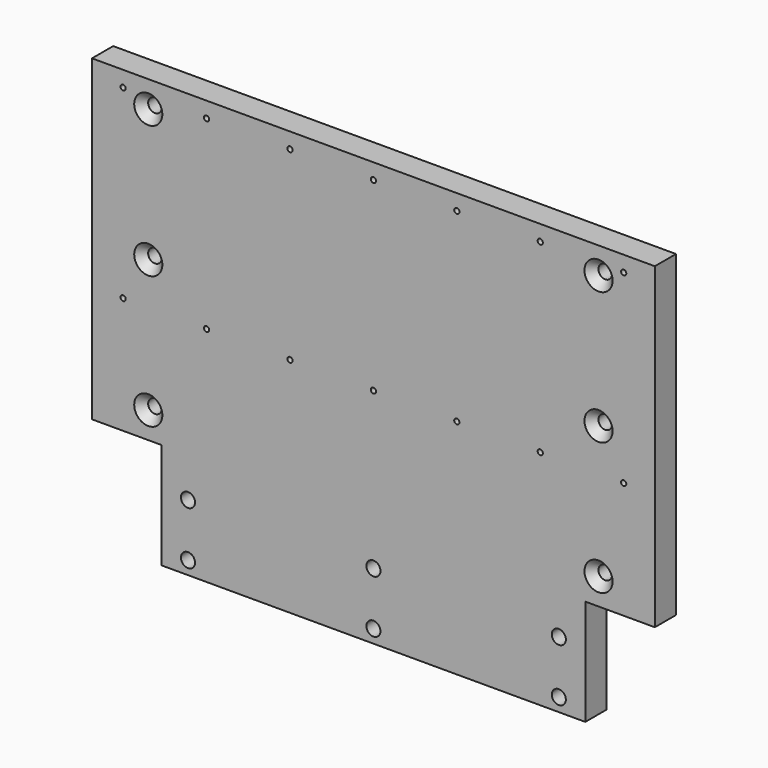
from build123d import *

# Parameters (mm, degrees)
F0_W           = 269.875
F0_H           = 203.2
F1_DEPTH       = 12.7
F2_W           = 33.3375
F2_H           = 50.8
F3_DEPTH       = 12.7
F5_D           = 6.7564
F7_D           = 2.5
F7_DEPTH       = 20.55
F7_TIP         = 0.7510757738
F9_D           = 6.5278
F9_CSINK_D     = 13.4874
F9_CSINK_ANGLE = 82


# Not quite as in the source:
# - a feature names something its author has since deleted; it is built from what else it names


with BuildPart() as f1:
    # F0 (on Front) → F1 (new body)
    with BuildSketch(Plane.XZ):
        with Locations((134.9375, 101.6)):
            Rectangle(F0_W, F0_H)
    extrude(amount=F1_DEPTH)

    # F2 (on face) → F3 (cut, through all)
    with BuildSketch(Plane.XZ.offset(12.7)):
        with Locations((16.66875, 25.4)):
            Rectangle(F2_W, F2_H)
        with Locations((253.20625, 25.4)):
            Rectangle(F2_W, F2_H)
    extrude(amount=-F3_DEPTH, mode=Mode.SUBTRACT)

    # F5 (through all)
    with Locations(Plane.XZ.offset(12.7)):
        with Locations((223.8375, 31.75), (223.8375, 6.35), (134.9375, 6.35), (134.9375, 31.75), (46.0375, 31.75), (46.0375, 6.35)):
            Hole(F5_D / 2)

    # F7
    with Locations(Plane.XZ.offset(12.7)):
        with Locations((54.9375, 195.7), (94.9375, 195.7), (134.9375, 195.7), (174.9375, 195.7), (214.9375, 195.7), (214.9375, 106.8), (174.9375, 106.8), (134.9375, 106.8), (94.9375, 106.8), (54.9375, 106.8), (14.9375, 195.7), (14.9375, 106.8), (254.9375, 195.7), (254.9375, 106.8)):
            Hole(F7_D / 2, depth=F7_DEPTH)
            with Locations((0, 0, -(F7_DEPTH + F7_TIP / 2))):  # 118° drill point
                Cone(0, F7_D / 2, F7_TIP, mode=Mode.SUBTRACT)

    # F9 (through all)
    with Locations(Plane.XZ.offset(12.7)):
        with Locations((26.9875, 190.5), (26.9875, 127), (26.9875, 63.5), (242.8875, 63.5), (242.8875, 127), (242.8875, 190.5)):
            CounterSinkHole(F9_D / 2, F9_CSINK_D / 2, counter_sink_angle=F9_CSINK_ANGLE)


solid = f1.part
